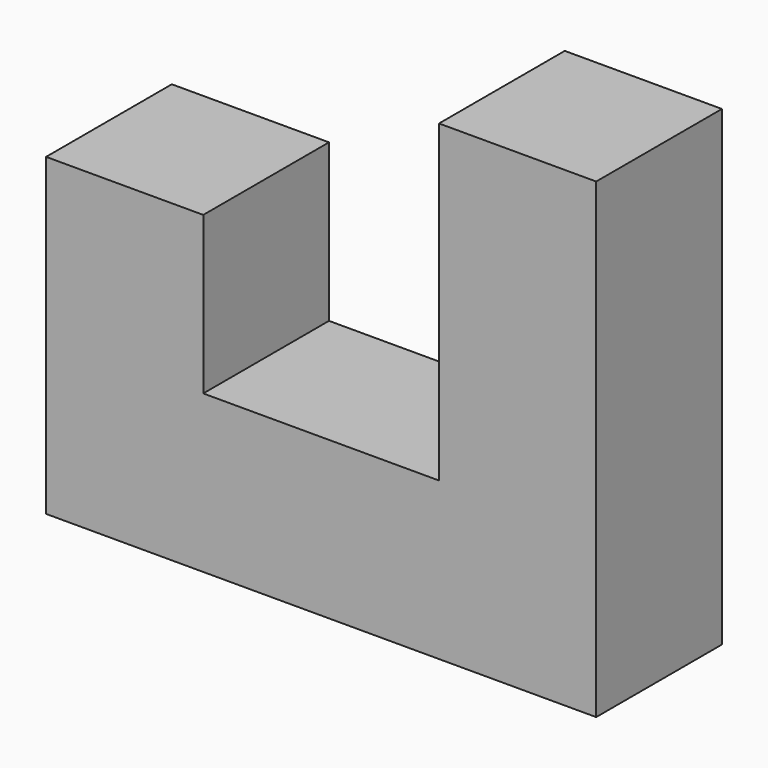
from build123d import *

# Parameters (mm, degrees)
F1_DEPTH = 25.4


# Not quite as in the source:
# - ends of sketch curves that miss each other by under 0.0002 mm in the source are joined


with BuildPart() as f1:
    # F0 (on Front) → F1 (new body)
    with BuildSketch(Plane.XZ):
        Polygon((-38.5571492787, -13.1272786043), (-38.5571492787, -63.9272786043), (50.3428467333, -63.9272786043), (50.3428467333, 12.2727213957), (24.9428467333, 12.2727213957), (24.9428467333, -38.5272786043), (-13.1571532667, -38.5272786043), (-13.1571532667, -13.1272786043), align=None)
    extrude(amount=-F1_DEPTH)


solid = f1.part
